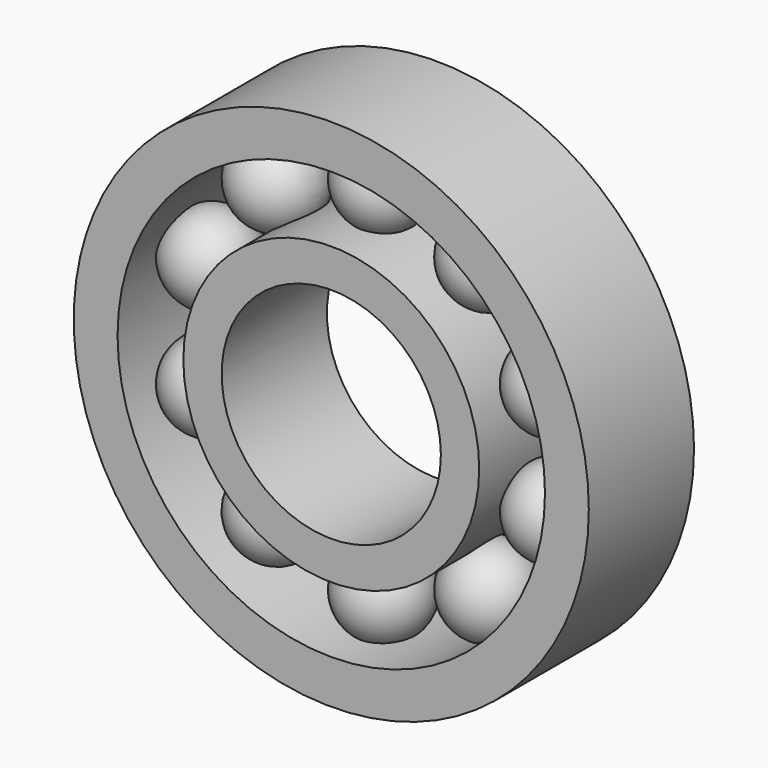
from build123d import *

# Parameters (mm, degrees)
F0_R     = 13.5
F0_R_2   = 10
F1_DEPTH = 6
F0_R_3   = 23.5
F0_R_4   = 19.5
F4_COUNT = 10


with BuildPart() as f1:
    # F0 (on Front) → F1 (new body, symmetric)
    with BuildSketch(Plane.XZ):
        Circle(F0_R)
        Circle(F0_R_2, mode=Mode.SUBTRACT)
    extrude(amount=F1_DEPTH, both=True)


with BuildPart() as f1b:
    # F0 (on Front) → F1, piece 2 (new body, symmetric)
    with BuildSketch(Plane.XZ):
        Circle(F0_R_3)
        Circle(F0_R_4, mode=Mode.SUBTRACT)
    extrude(amount=F1_DEPTH, both=True)


with BuildPart() as f3:
    # F2 (on Front) → F3 (revolve)
    with BuildSketch(Plane.XZ):
        with BuildLine():
            Line((0, 20.5), (0, 12.5))
            ThreePointArc((0, 12.5), (4, 16.5), (0, 20.5))
        make_face()
    revolve(axis=Axis((0, 0, 16.5), (0, 0, -1)))


with BuildPart() as f4_1:
    # F4: instance of F3
    add(f3.part.rotate(Axis((0, 0, 0), (0, -1, 0)), 1 * 360 / F4_COUNT))


with BuildPart() as f4_2:
    # F4: instance of F3
    add(f3.part.rotate(Axis((0, 0, 0), (0, -1, 0)), 2 * 360 / F4_COUNT))


with BuildPart() as f4_3:
    # F4: instance of F3
    add(f3.part.rotate(Axis((0, 0, 0), (0, -1, 0)), 3 * 360 / F4_COUNT))


with BuildPart() as f4_4:
    # F4: instance of F3
    add(f3.part.rotate(Axis((0, 0, 0), (0, -1, 0)), 4 * 360 / F4_COUNT))


with BuildPart() as f4_5:
    # F4: instance of F3
    add(f3.part.rotate(Axis((0, 0, 0), (0, -1, 0)), 5 * 360 / F4_COUNT))


with BuildPart() as f4_6:
    # F4: instance of F3
    add(f3.part.rotate(Axis((0, 0, 0), (0, -1, 0)), 6 * 360 / F4_COUNT))


with BuildPart() as f4_7:
    # F4: instance of F3
    add(f3.part.rotate(Axis((0, 0, 0), (0, -1, 0)), 7 * 360 / F4_COUNT))


with BuildPart() as f4_8:
    # F4: instance of F3
    add(f3.part.rotate(Axis((0, 0, 0), (0, -1, 0)), 8 * 360 / F4_COUNT))


with BuildPart() as f4_9:
    # F4: instance of F3
    add(f3.part.rotate(Axis((0, 0, 0), (0, -1, 0)), 9 * 360 / F4_COUNT))


solid = Compound([f1.part, f1b.part, f3.part, f4_1.part, f4_2.part, f4_3.part, f4_4.part, f4_5.part, f4_6.part, f4_7.part, f4_8.part, f4_9.part])
